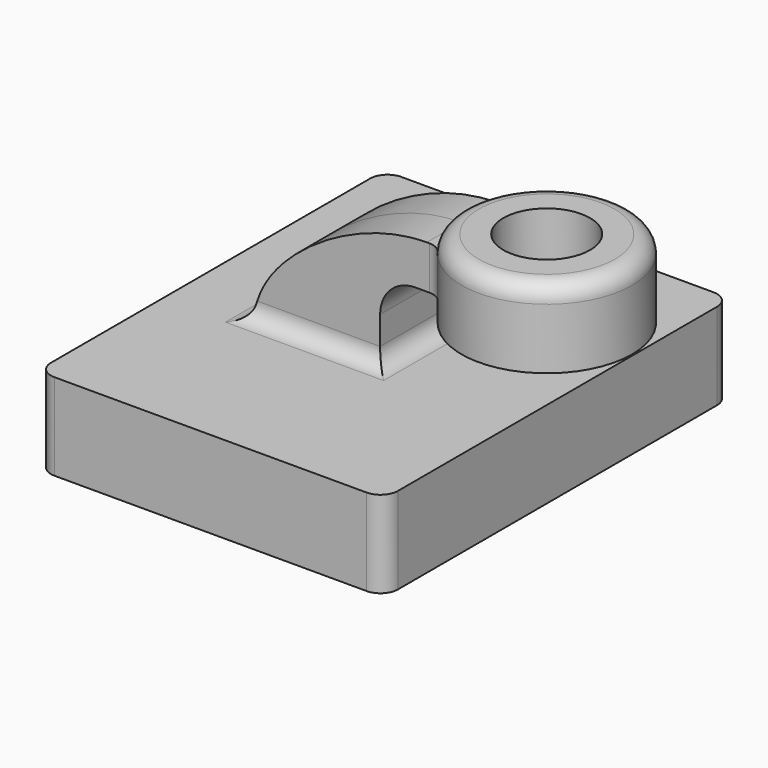
from build123d import *

# Parameters (mm, degrees)
F1_DEPTH  = 63.5
F2_DEPTH  = 63.5
F3_DEPTH  = 12.7
F5_R      = 5.08
F6_R      = 5.08
F7_R      = 5.07999
F10_D     = 25.4
F10_DEPTH = 22.8609980474


# Not quite as in the source:
# - a fillet or chamfer is up to 0.001 mm smaller than in the source, because OpenCascade refuses the exact size


with BuildPart() as f1:
    # F0 (on Front) → F1 (new body, symmetric)
    with BuildSketch(Plane.XZ):
        Polygon((-27.7423580625, 12.7), (-50.8, 12.7), (-50.8, -12.7), (50.8, -12.7), (50.8, 12.7), (9.0188104659, 12.7), align=None)
    extrude(amount=F1_DEPTH, both=True)

    # F0 (on Front) → F2 (join, symmetric)
    with BuildSketch(Plane.XZ):
        Polygon((-27.7423580625, 12.7), (-50.8, 12.7), (-50.8, -12.7), (50.8, -12.7), (50.8, 12.7), (9.0188104659, 12.7), align=None)
    extrude(amount=F2_DEPTH, both=True)

    # F0 (on Front) → F3 (join, symmetric)
    with BuildSketch(Plane.XZ):
        with BuildLine():
            add(Edge.make_bspline(
                [(-27.7423580625, 12.7), (-27.7423580625, 29.5749301373), (-0.0054883666, 49.0460789908), (22.6876754314, 49.0499310609)],
                knots=[0, 0, 0, 0, 62.1644632252, 62.1644632252, 62.1644632252, 62.1644632252], degree=3))
            Line((-27.7423580625, 12.7), (9.0188104659, 12.7))
            Line((9.0188104659, 12.7), (9.0188104659, 26.0071345331))
            ThreePointArc((9.0188104659, 26.0071345331), (12.0481455999, 33.3205964986), (19.3616075654, 36.3499316326))
            Line((19.3616075654, 36.3499316326), (22.6876754314, 36.3499316326))
            Line((22.6876754314, 36.3499316326), (22.6876754314, 49.0499310609))
        make_face()
        with BuildLine():
            add(Edge.make_bspline(
                [(22.6876754314, 49.0499310609), (22.689920498, 49.049931442), (22.6921655153, 49.0499316326), (22.6944104832, 49.0499316326)],
                knots=[62.1644632252, 62.1644632252, 62.1644632252, 62.1644632252, 62.1706132431, 62.1706132431, 62.1706132431, 62.1706132431], degree=3))
            Line((22.6876754314, 49.0499310609), (22.6876754314, 36.3499316326))
            Line((22.6876754314, 36.3499316326), (47.668707557, 36.3499316326))
            Line((47.668707557, 36.3499316326), (47.668707557, 49.0499316326))
            Line((47.668707557, 49.0499316326), (22.6944104832, 49.0499316326))
        make_face()
    extrude(amount=F3_DEPTH, both=True)

    # F0 (on Front) → F4 (revolve)
    with BuildSketch(Plane.XZ):
        Polygon((72.6497396827, 54.1299306562), (47.668707557, 54.1299306562), (47.668707557, 49.0499316326), (47.668707557, 36.3499316326), (47.668707557, 31.2699326089), (72.6497396827, 31.2699326089), align=None)
    revolve(axis=Axis((47.668707557, 0, 42.6999316326), (0, 0, -1)))

    # F5
    f5_edges = [f1.edges().sort_by_distance(p)[0] for p in [
        (-9.361774, -12.7, 12.7),
        (9.01881, 0, 12.7),
        (-27.742358, 6.35, 12.7),
        (-27.742358, -6.35, 12.7),
        (-9.361774, 12.7, 12.7),
        (-50.8, -63.5, 0),
        (-50.8, 63.5, 0),
        (50.8, -63.5, 0),
        (50.8, 63.5, 0),
    ]]
    fillet(f5_edges, radius=F5_R)

    # F6
    f6_edges = [f1.edges().sort_by_distance(p)[0] for p in [
        (26.156805, -12.7, 42.699932),
        (26.156805, 12.7, 42.699932),
    ]]
    fillet(f6_edges, radius=F6_R)

    # F7 (radius 5.08 in the source; OpenCascade refuses exactly that, so slightly less here)
    f7_edges = [f1.edges().sort_by_distance(p)[0] for p in [
        (22.687675, 0, 54.129931),
    ]]
    fillet(f7_edges, radius=F7_R)

    # F10 (through all, one way)
    with BuildSketch(Plane(origin=(0, 0, 31.2699326089), x_dir=(1, 0, 0), z_dir=(0, 0, -1))):
        with Locations((47.61569947, -0.0454496221)):
            Circle(F10_D / 2)
    extrude(amount=-F10_DEPTH, mode=Mode.SUBTRACT)


solid = f1.part
